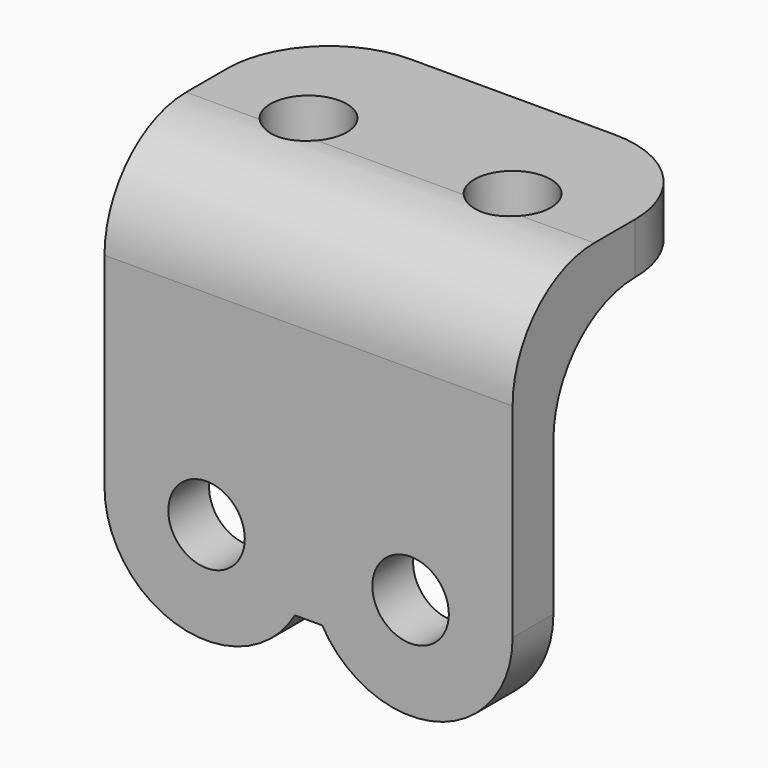
from build123d import *

# Parameters (mm, degrees)
F1_DEPTH     = 25.4
F2_R         = 2.38125
F3_DEPTH     = 28.576
F4_R         = 2.38125
F5_DEPTH     = 15.876
F6_T4_DEPTH  = 25.4
F6_S5_R      = 2.38125
F6_T6_DEPTH  = 15
F6_S7_R      = 2.38125
F6_T8_DEPTH  = 15
F6_T9_DEPTH  = 57.15
F6_T11_DEPTH = 34.925


# Not quite as in the source:
# - a fillet or chamfer that OpenCascade refuses, or shapes differently, is made with other operations: its cross-section is extruded or revolved along the edge and cut away or added


with BuildPart() as f1:
    # F0 (on Right) → F1 (new body)
    with BuildSketch(Plane.YZ):
        Polygon((0, 0), (12.7, 0), (12.7, 3.175), (-3.175, 3.175), (-3.175, -25.4), (0, -25.4), align=None)
    extrude(amount=F1_DEPTH)

    # F2 (on face) → F3 (cut, through all)
    with BuildSketch(Plane.XY.offset(3.175)):
        with Locations((6.35, 4.7625)):
            Circle(F2_R)
        with Locations((19.05, 4.7625)):
            Circle(F2_R)
    extrude(amount=-F3_DEPTH, mode=Mode.SUBTRACT)

    # F4 (on face) → F5 (cut, through all)
    with BuildSketch(Plane.XZ.offset(3.175)):
        with BuildLine():
            Line((13.550738686, -19.05), (11.849261314, -19.05))
            ThreePointArc((11.849261314, -19.05), (4.706499047, -22.0086289925), (0, -15.8749999656))
            Line((0, -15.8749999656), (0, -25.4))
            Line((0, -25.4), (25.4, -25.4))
            Line((25.4, -25.4), (25.4, -15.875))
            ThreePointArc((25.4, -15.875), (20.6935009364, -22.0086289969), (13.550738686, -19.05))
        make_face()
        with Locations((19.05, -15.875)):
            Circle(F4_R)
        with Locations((6.35, -15.875)):
            Circle(F4_R)
    extrude(amount=-F5_DEPTH, mode=Mode.SUBTRACT)

    # F6: fillet of radius 6.35 on 4 edges, made by hand


with BuildPart() as f6_tool2:
    # F6_s3 → F6_t4 (new body)
    with BuildSketch(Plane.YZ):
        with BuildLine():
            ThreePointArc((6.35, 0), (1.8598719395, -1.8598719395), (0, -6.35))
            Line((0, -6.35), (0, 0))
            Line((0, 0), (6.35, 0))
        make_face()
    extrude(amount=F6_T4_DEPTH)

    # F6_s5 → F6_t6 (cut, symmetric)
    with BuildSketch(Plane.XY.offset(-3.2)):
        with Locations((19.05, 4.7625)):
            Circle(F6_S5_R)
    extrude(amount=F6_T6_DEPTH, both=True, mode=Mode.SUBTRACT)

    # F6_s7 → F6_t8 (cut, symmetric)
    with BuildSketch(Plane.XY.offset(-3.2)):
        with Locations((6.35, 4.7625)):
            Circle(F6_S7_R)
    extrude(amount=F6_T8_DEPTH, both=True, mode=Mode.SUBTRACT)


with BuildPart() as f1_1:
    add(f1.part)

    # F6_t1: union F6_tool2
    add(f6_tool2.part)

    # F6_s10 → F6_t9 (cut)
    with BuildSketch(Plane.YZ.offset(-15.875)):
        with BuildLine():
            ThreePointArc((3.175, 3.175), (-1.3151280605, 1.3151280605), (-3.175, -3.175))
            Line((-3.175, -3.175), (-3.175, 3.175))
            Line((-3.175, 3.175), (3.175, 3.175))
        make_face()
    extrude(amount=F6_T9_DEPTH, mode=Mode.SUBTRACT)

    # F6_s12 → F6_t11 (cut)
    with BuildSketch(Plane.XY.offset(-15.875)):
        with BuildLine():
            ThreePointArc((6.35, 12.7), (1.8598719395, 10.8401280605), (0, 6.35))
            Line((0, 6.35), (0, 12.7))
            Line((0, 12.7), (6.35, 12.7))
        make_face()
        with BuildLine():
            ThreePointArc((25.4, 6.35), (23.5401280605, 10.8401280605), (19.05, 12.7))
            Line((19.05, 12.7), (25.4, 12.7))
            Line((25.4, 12.7), (25.4, 6.35))
        make_face()
    extrude(amount=F6_T11_DEPTH, mode=Mode.SUBTRACT)


solid = f1_1.part
